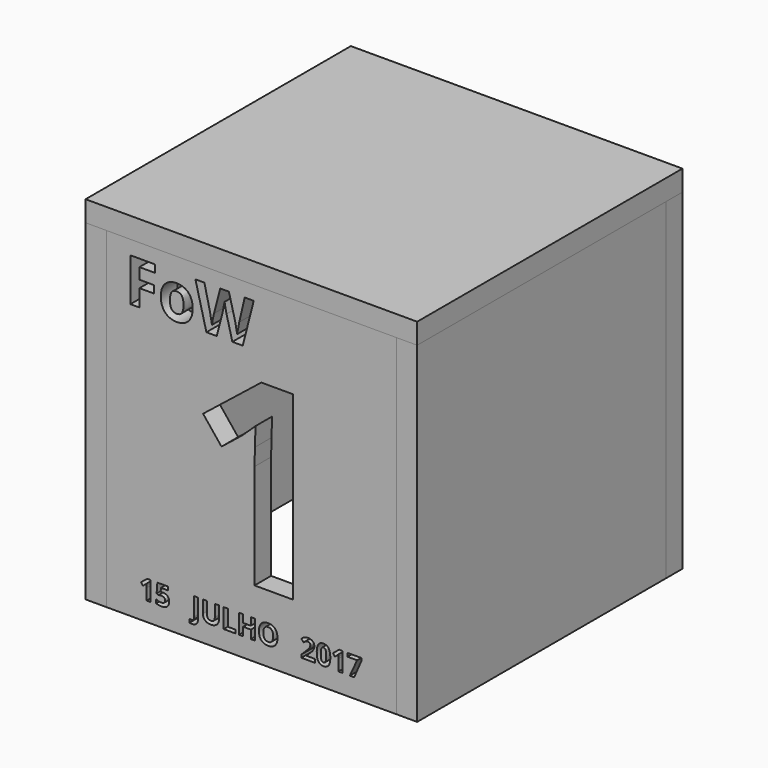
from build123d import *

# Parameters (mm, degrees)
F0_W            = 40
F0_H            = 40
F1_DEPTH        = 2.5
F2_W            = 40
F2_H            = 40
F3_DEPTH        = 2.5
F4_W            = 40
F4_H            = 40
F5_DEPTH        = 2.5
F6_W            = 40
F6_H            = 40
F7_DEPTH        = 2.5
F8_W            = 40
F8_H            = 40
F9_DEPTH        = 2.5
F10_TEXT_SIZE   = 7.2732438383
F10_TEXT_SIZE_2 = 30.5555555556
F10_TEXT_SIZE_3 = 3.2806804374
F11_DEPTH       = 3


# Not quite as in the source:
# - Text() gives the source's letters only with a copy of the font that has no kerning and outlines rounded to 1/6400 em; it was checked with that copy


with BuildPart() as f1:
    # F0 (on Top) → F1 (new body)
    with BuildSketch(Plane.XY):
        with Locations((-20, 20)):
            Rectangle(F0_W, F0_H)
    extrude(amount=F1_DEPTH)


with BuildPart() as f3:
    # F2 (on face) → F3 (new body)
    with BuildSketch(Plane.XZ):
        with Locations((-20, -20)):
            Rectangle(F2_W, F2_H)
    extrude(amount=-F3_DEPTH)

    # F10 (on face) → F11 (cut)
    with BuildSketch(Plane.XZ):
        with Locations((-35.2436941774, -6.8869412126)):
            Text('FoW', F10_TEXT_SIZE, font='Open Sans', font_style=FontStyle.BOLD, text_align=(TextAlign.LEFT, TextAlign.BOTTOM))
        with Locations((-27.6295324308, -31.8866075277)):
            Text('1', F10_TEXT_SIZE_2, font='Open Sans', font_style=FontStyle.BOLD, text_align=(TextAlign.LEFT, TextAlign.BOTTOM))
        with Locations((-33.5055664182, -37.734027952)):
            Text('15   JULHO   2017', F10_TEXT_SIZE_3, font='Open Sans', font_style=FontStyle.BOLD, text_align=(TextAlign.LEFT, TextAlign.BOTTOM))
    extrude(amount=-F11_DEPTH, mode=Mode.SUBTRACT)


with BuildPart() as f5:
    # F4 (on face) → F5 (new body)
    with BuildSketch(Plane.YZ):
        with Locations((20, -20)):
            Rectangle(F4_W, F4_H)
    extrude(amount=-F5_DEPTH)


with BuildPart() as f7:
    # F6 (on face) → F7 (new body)
    with BuildSketch(Plane(origin=(0, 40, 0), x_dir=(-1, 0, 0), z_dir=(0, 1, 0))):
        with Locations((20, -20)):
            Rectangle(F6_W, F6_H)
    extrude(amount=-F7_DEPTH)


with BuildPart() as f9:
    # F8 (on face) → F9 (new body)
    with BuildSketch(Plane(origin=(-40, 0, 0), x_dir=(0, -1, 0), z_dir=(-1, 0, 0))):
        with Locations((-20, -20)):
            Rectangle(F8_W, F8_H)
    extrude(amount=-F9_DEPTH)


solid = Compound([f1.part, f3.part, f5.part, f7.part, f9.part])
